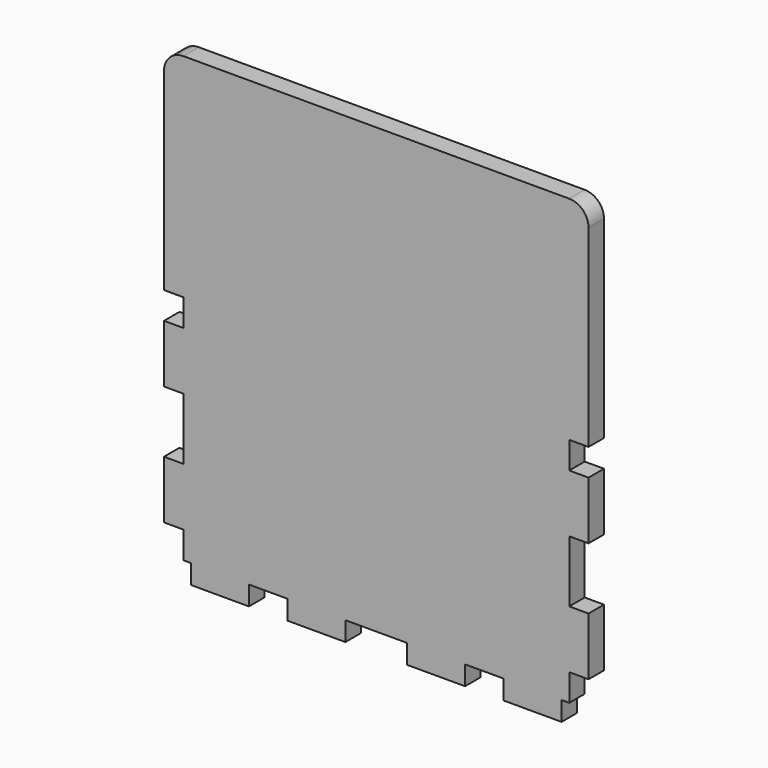
from build123d import *

# Parameters (mm, degrees)
F1_DEPTH = 5
F2_DEPTH = 5
F3_DEPTH = 5


# Not quite as in the source:
# - a feature names something its author has since deleted; it is built from what else it names


with BuildPart() as f1:
    # F0 (on Front) → F1 (new body)
    with BuildSketch(Plane.XZ):
        Polygon((-50.9245342757, -5.52e-08), (-100.9245342757, -5.52e-08), (-100.9245342757, -7), (-105.9245342757, -7), (-105.924534339, -22), (-100.9245342757, -22), (-100.9245342757, -38), (-105.9245342757, -38), (-105.924534339, -53), (-100.9245342757, -53), (-100.9245342757, -60.0000000552), (-98.924534339, -60.0000000552), (-98.924534339, -65.0000000552), (-83.924534339, -65), (-83.924534339, -60.0000000552), (-73.924534339, -60.0000000552), (-73.924534339, -65.0000000552), (-58.924534339, -65), (-58.924534339, -60.0000000552), (-42.9245342757, -60.0000000552), (-42.9245342757, -65.0000000552), (-27.9245342757, -65.0000000552), (-27.9245342757, -60.0000000552), (-17.9245342757, -60.0000000552), (-17.9245342757, -65.0000000552), (-2.9245342757, -65.0000000552), (-2.9245342757, -60.0000000552), (-0.9245342757, -60.0000000552), (-0.9245342757, -53.0000000552), (4.0754657243, -53.0000000552), (4.0754657243, -38.0000000552), (-0.9245342757, -38.0000000552), (-0.9245342757, -22), (4.0754657243, -22), (4.075465661, -7), (-0.9245342757, -7), (-0.9245342757, -5.52e-08), align=None)
    extrude(amount=F1_DEPTH)

    # F0 (on Front) → F2 (join)
    with BuildSketch(Plane.XZ):
        with BuildLine():
            Line((-105.9245342757, -5.52e-08), (-100.9245342757, -5.52e-08))
            Line((-100.9245342757, -5.52e-08), (-50.9245342757, -5.52e-08))
            Line((-50.9245342757, -5.52e-08), (-0.9245342757, -5.52e-08))
            Line((-0.9245342757, -5.52e-08), (4.0754657243, -5.52e-08))
            Line((4.0754657243, -5.52e-08), (4.0754657243, 49.9999999448))
            ThreePointArc((4.0754657243, 49.9999999448), (2.6109996302, 53.5355338508), (-0.9245342757, 54.9999999448))
            Line((-0.9245342757, 54.9999999448), (-100.9245342757, 54.9999999448))
            ThreePointArc((-100.9245342757, 54.9999999448), (-104.4600681817, 53.5355338508), (-105.9245342757, 49.9999999448))
            Line((-105.9245342757, 49.9999999448), (-105.9245342757, -5.52e-08))
        make_face()
    extrude(amount=F2_DEPTH)

    # F0 (on Front) → F3 (join)
    with BuildSketch(Plane.XZ):
        with BuildLine():
            Line((-105.9245342757, -5.52e-08), (-100.9245342757, -5.52e-08))
            Line((-100.9245342757, -5.52e-08), (-50.9245342757, -5.52e-08))
            Line((-50.9245342757, -5.52e-08), (-0.9245342757, -5.52e-08))
            Line((-0.9245342757, -5.52e-08), (4.0754657243, -5.52e-08))
            Line((4.0754657243, -5.52e-08), (4.0754657243, 49.9999999448))
            ThreePointArc((4.0754657243, 49.9999999448), (2.6109996302, 53.5355338508), (-0.9245342757, 54.9999999448))
            Line((-0.9245342757, 54.9999999448), (-100.9245342757, 54.9999999448))
            ThreePointArc((-100.9245342757, 54.9999999448), (-104.4600681817, 53.5355338508), (-105.9245342757, 49.9999999448))
            Line((-105.9245342757, 49.9999999448), (-105.9245342757, -5.52e-08))
        make_face()
    extrude(amount=F3_DEPTH)


solid = f1.part
